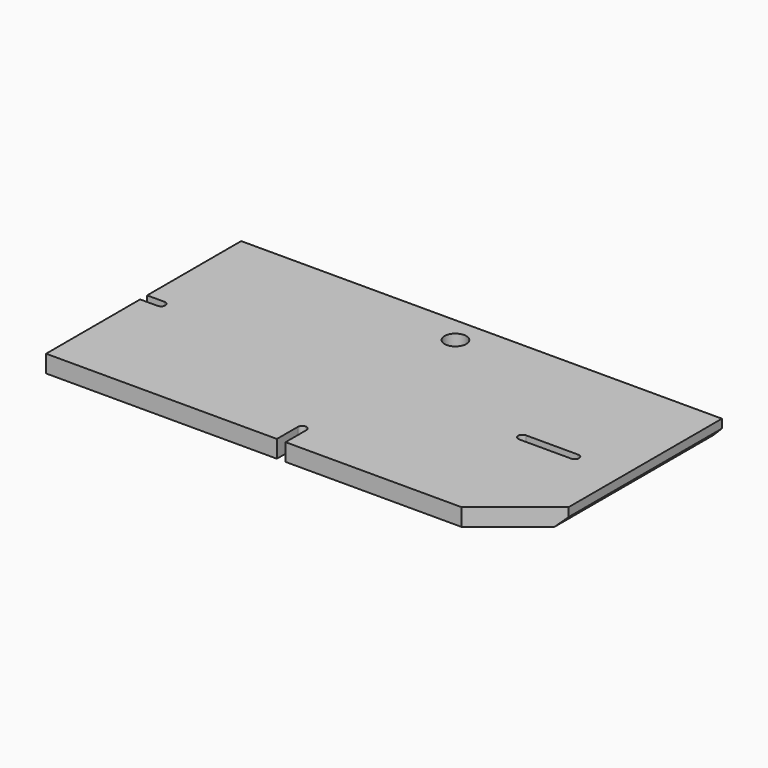
from build123d import *

# Parameters (mm, degrees)
F1_DEPTH = 25.4
F2_W     = 31.75
F2_H     = 12.7
F2_W_2   = 88.9
F2_R     = 15.875
F3_DEPTH = 25.401
F4_R     = 6.34999
F5_SIZE  = 12.7


# Not quite as in the source:
# - a fillet or chamfer is up to 0.001 mm smaller than in the source, because OpenCascade refuses the exact size


with BuildPart() as f1:
    # F0 (on Top) → F1 (new body)
    with BuildSketch(Plane.XY):
        Polygon((-50.9642694569, 222.8586515407), (-409.1042694569, 222.8586515407), (-409.1042694569, 57.7525011744), (-409.1042694569, 32.4011304667), (-409.1042694569, -132.7413484593), (196.6857305431, -132.7413484593), (291.9357305431, -56.5413484593), (291.9357305431, 222.8586515407), (-49.417052418, 222.8586515407), align=None)
    extrude(amount=F1_DEPTH)

    # F2 (on face) → F3 (cut, through all)
    with BuildSketch(Plane.XY.offset(25.4)):
        with Locations((-393.2292694569, 45.0586515407)):
            Rectangle(F2_W, F2_H)
        with Locations((181.4457305431, 45.0586515407)):
            Rectangle(F2_W_2, F2_H)
        with BuildLine():
            Line((-59.8542694569, -142.5310963776), (-59.8542694569, -94.6413484593))
            ThreePointArc((-59.8542694569, -94.6413484593), (-66.2042694569, -88.2913484593), (-72.5542694569, -94.6413484593))
            Line((-72.5542694569, -94.6413484593), (-72.5542694569, -137.446552515))
            Line((-72.5542694569, -137.446552515), (-59.8542694569, -142.5310963776))
        make_face()
        with Locations((-66.2042694569, 184.7586515407)):
            Circle(F2_R)
    extrude(amount=-F3_DEPTH, mode=Mode.SUBTRACT)

    # F4 (radius 6.35 in the source; OpenCascade refuses exactly that, so slightly less here)
    f4_edges = [f1.edges().sort_by_distance(p)[0] for p in [
        (-377.354269, 51.408652, 12.7),
        (225.895731, 51.408652, 12.7),
        (225.895731, 38.708652, 12.7),
        (-377.354269, 38.708652, 12.7),
        (136.995731, 51.408652, 12.7),
        (136.995731, 38.708652, 12.7),
    ]]
    fillet(f4_edges, radius=F4_R)

    # F5
    f5_edges = [f1.edges().sort_by_distance(p)[0] for p in [
        (291.935731, 83.158652, 0),
    ]]
    chamfer(f5_edges, length=F5_SIZE)


solid = f1.part
